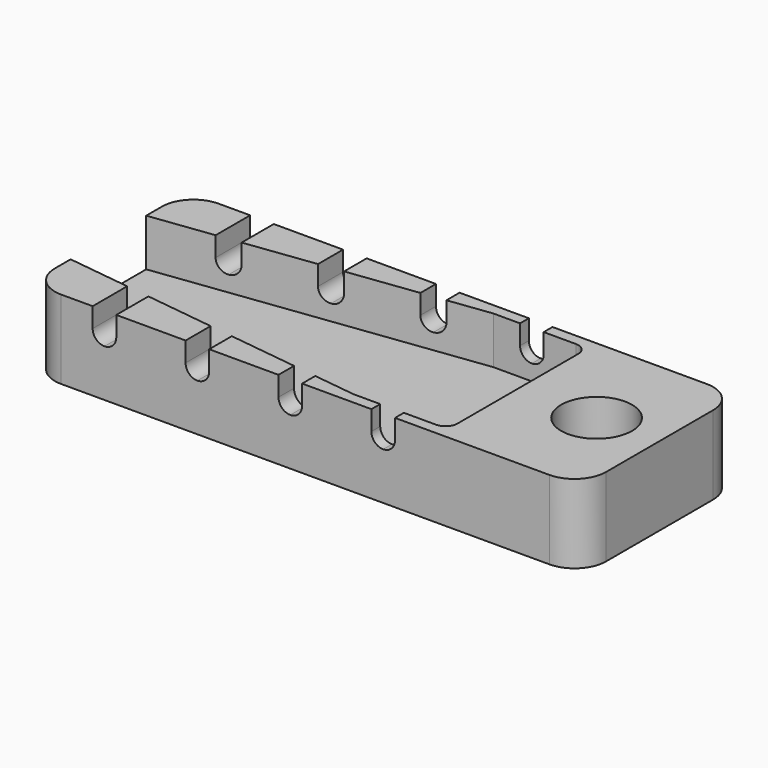
from build123d import *

# Parameters (mm, degrees)
F0_W     = 1.5
F0_H     = 0.7
F0_R     = 2.25
F0_H_2   = 11.1
F0_W_2   = 2.8
F1_DEPTH = 5
F2_DEPTH = 3
F3_DEPTH = 2
F4_R     = 0.74999
F5_R     = 2


# Not quite as in the source:
# - a fillet or chamfer is up to 0.001 mm smaller than in the source, because OpenCascade refuses the exact size


with BuildPart() as f1:
    # F0 (on Top) → F1 (new body)
    with BuildSketch(Plane.XY):
        Polygon((-18.8879279066, 6.25), (-22.8879279066, 6.25), (-22.8879279066, 3), (-18.8879279066, 3.51), align=None)
        Polygon((-17.3879279066, 6.25), (-18.8879279066, 6.25), (-18.8879279066, 3.51), (-17.3879279066, 3.70125), align=None)
        Polygon((-18.8879279066, 3.51), (-22.8879279066, 3), (-22.8879279066, -3), (-18.8879279066, -3.51), align=None)
        Polygon((-12.9879279066, 6.25), (-17.3879279066, 6.25), (-17.3879279066, 3.70125), (-12.9879279066, 4.26225), align=None)
        Polygon((-18.8879279066, -3.51), (-22.8879279066, -3), (-22.8879279066, -6.25), (-18.8879279066, -6.25), align=None)
        Polygon((-11.4879279066, 6.25), (-12.9879279066, 6.25), (-12.9879279066, 4.26225), (-11.4879279066, 4.4535), align=None)
        Polygon((-17.3879279066, -3.70125), (-18.8879279066, -3.51), (-18.8879279066, -6.25), (-17.3879279066, -6.25), align=None)
        Polygon((-7.0879279066, 6.25), (-11.4879279066, 6.25), (-11.4879279066, 4.4535), (-7.0879279066, 5.0145), align=None)
        Polygon((-12.9879279066, -4.26225), (-17.3879279066, -3.70125), (-17.3879279066, -6.25), (-12.9879279066, -6.25), align=None)
        Polygon((-5.5879279066, 6.25), (-7.0879279066, 6.25), (-7.0879279066, 5.0145), (-5.5879279066, 5.20575), align=None)
        Polygon((-11.4879279066, -4.4535), (-12.9879279066, -4.26225), (-12.9879279066, -6.25), (-11.4879279066, -6.25), align=None)
        Polygon((-1.1879279066, 6.25), (-5.5879279066, 6.25), (-5.5879279066, 5.20575), (-2.8879279066, 5.55), (-1.1879279066, 5.55), align=None)
        Polygon((-7.0879279066, -5.0145), (-11.4879279066, -4.4535), (-11.4879279066, -6.25), (-7.0879279066, -6.25), align=None)
        with Locations((-0.4379279066, 5.9)):
            Rectangle(F0_W, F0_H)
        Polygon((-5.5879279066, -5.20575), (-7.0879279066, -5.0145), (-7.0879279066, -6.25), (-5.5879279066, -6.25), align=None)
        Polygon((12.1120720934, 6.25), (0.3120720934, 6.25), (0.3120720934, 5.55), (3.1120720934, 5.55), (3.1120720934, -5.55), (0.3120720934, -5.55), (0.3120720934, -6.25), (12.1120720934, -6.25), align=None)
        with Locations((8.1120720934, 0)):
            Circle(F0_R, mode=Mode.SUBTRACT)
        Polygon((-2.8879279066, -5.55), (-5.5879279066, -5.20575), (-5.5879279066, -6.25), (-1.1879279066, -6.25), (-1.1879279066, -5.55), align=None)
        with Locations((-0.4379279066, -5.9)):
            Rectangle(F0_W, F0_H)
        with Locations((-0.4379279066, 0)):
            Rectangle(F0_W, F0_H_2)
        Polygon((-5.5879279066, 5.20575), (-7.0879279066, 5.0145), (-7.0879279066, -5.0145), (-5.5879279066, -5.20575), align=None)
        Polygon((-17.3879279066, 3.70125), (-18.8879279066, 3.51), (-18.8879279066, -3.51), (-17.3879279066, -3.70125), align=None)
        Polygon((-12.9879279066, 4.26225), (-17.3879279066, 3.70125), (-17.3879279066, -3.70125), (-12.9879279066, -4.26225), align=None)
        Polygon((-7.0879279066, 5.0145), (-11.4879279066, 4.4535), (-11.4879279066, -4.4535), (-7.0879279066, -5.0145), align=None)
        Polygon((-11.4879279066, 4.4535), (-12.9879279066, 4.26225), (-12.9879279066, -4.26225), (-11.4879279066, -4.4535), align=None)
        Polygon((-2.8879279066, 5.55), (-5.5879279066, 5.20575), (-5.5879279066, -5.20575), (-2.8879279066, -5.55), (-1.1879279066, -5.55), (-1.1879279066, 5.55), align=None)
        with Locations((1.7120720934, 0)):
            Rectangle(F0_W_2, F0_H_2)
    extrude(amount=-F1_DEPTH)

    # F0 (on Top) → F2 (cut)
    with BuildSketch(Plane.XY):
        Polygon((-18.8879279066, 3.51), (-22.8879279066, 3), (-22.8879279066, -3), (-18.8879279066, -3.51), align=None)
        Polygon((-17.3879279066, 3.70125), (-18.8879279066, 3.51), (-18.8879279066, -3.51), (-17.3879279066, -3.70125), align=None)
        Polygon((-12.9879279066, 4.26225), (-17.3879279066, 3.70125), (-17.3879279066, -3.70125), (-12.9879279066, -4.26225), align=None)
        Polygon((-11.4879279066, 4.4535), (-12.9879279066, 4.26225), (-12.9879279066, -4.26225), (-11.4879279066, -4.4535), align=None)
        Polygon((-7.0879279066, 5.0145), (-11.4879279066, 4.4535), (-11.4879279066, -4.4535), (-7.0879279066, -5.0145), align=None)
        Polygon((-5.5879279066, 5.20575), (-7.0879279066, 5.0145), (-7.0879279066, -5.0145), (-5.5879279066, -5.20575), align=None)
        Polygon((-2.8879279066, 5.55), (-5.5879279066, 5.20575), (-5.5879279066, -5.20575), (-2.8879279066, -5.55), (-1.1879279066, -5.55), (-1.1879279066, 5.55), align=None)
        with Locations((-0.4379279066, 0)):
            Rectangle(F0_W, F0_H_2)
        with Locations((1.7120720934, 0)):
            Rectangle(F0_W_2, F0_H_2)
    extrude(amount=-F2_DEPTH, mode=Mode.SUBTRACT)

    # F0 (on Top) → F3 (cut)
    with BuildSketch(Plane.XY):
        Polygon((-17.3879279066, 6.25), (-18.8879279066, 6.25), (-18.8879279066, 3.51), (-17.3879279066, 3.70125), align=None)
        Polygon((-11.4879279066, 6.25), (-12.9879279066, 6.25), (-12.9879279066, 4.26225), (-11.4879279066, 4.4535), align=None)
        Polygon((-5.5879279066, 6.25), (-7.0879279066, 6.25), (-7.0879279066, 5.0145), (-5.5879279066, 5.20575), align=None)
        with Locations((-0.4379279066, -5.9)):
            Rectangle(F0_W, F0_H)
        Polygon((-17.3879279066, -3.70125), (-18.8879279066, -3.51), (-18.8879279066, -6.25), (-17.3879279066, -6.25), align=None)
        Polygon((-11.4879279066, -4.4535), (-12.9879279066, -4.26225), (-12.9879279066, -6.25), (-11.4879279066, -6.25), align=None)
        Polygon((-5.5879279066, -5.20575), (-7.0879279066, -5.0145), (-7.0879279066, -6.25), (-5.5879279066, -6.25), align=None)
        with Locations((-0.4379279066, 5.9)):
            Rectangle(F0_W, F0_H)
    extrude(amount=-F3_DEPTH, mode=Mode.SUBTRACT)

    # F4 (radius 0.75 in the source; OpenCascade refuses exactly that, so slightly less here)
    f4_edges = [f1.edges().sort_by_distance(p)[0] for p in [
        (-17.387928, -4.975625, -2),
        (-11.487928, -5.35175, -2),
        (-5.587928, -5.727875, -2),
        (0.312072, -5.9, -2),
        (-18.887928, -4.88, -2),
        (-12.987928, -5.256125, -2),
        (-7.087928, -5.63225, -2),
        (-1.187928, -5.9, -2),
        (-18.887928, 4.88, -2),
        (-12.987928, 5.256125, -2),
        (-7.087928, 5.63225, -2),
        (-1.187928, 5.9, -2),
        (-17.387928, 4.975625, -2),
        (-11.487928, 5.35175, -2),
        (-5.587928, 5.727875, -2),
        (0.312072, 5.9, -2),
        (3.112072, 5.55, -1.5),
        (3.112072, -5.55, -1.5),
    ]]
    fillet(f4_edges, radius=F4_R)

    # F5
    f5_edges = [f1.edges().sort_by_distance(p)[0] for p in [
        (-22.887928, -6.25, -2.5),
        (-22.887928, 6.25, -2.5),
        (12.112072, -6.25, -2.5),
        (12.112072, 6.25, -2.5),
    ]]
    fillet(f5_edges, radius=F5_R)


solid = f1.part
